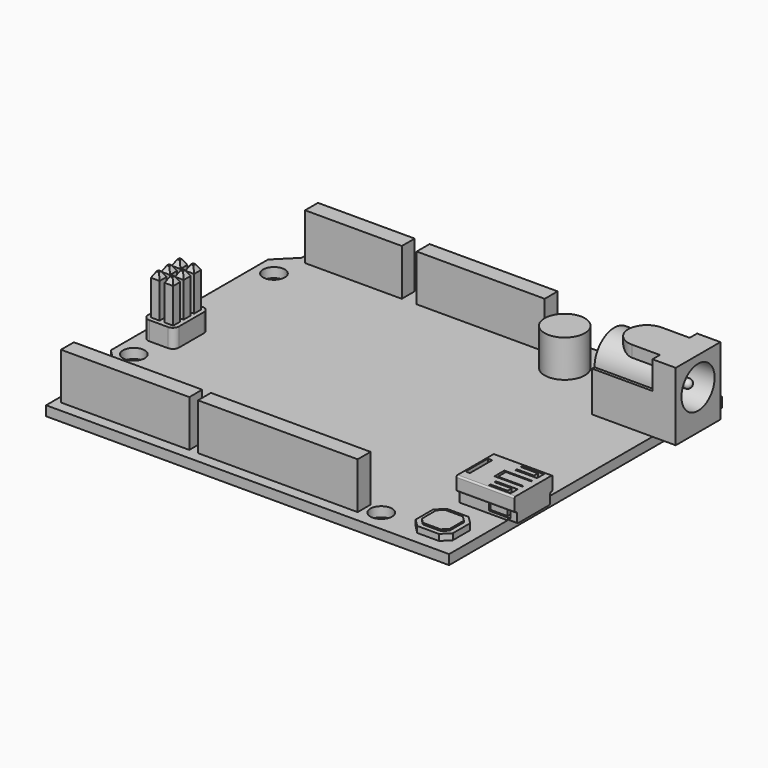
from build123d import *

# Parameters (mm, degrees)
F0_W           = 65
F0_H           = 55
F1_DEPTH       = 1.57
F3_DEPTH       = 1.57
F4_R           = 1.75
F5_DEPTH       = 1.571
F6_W           = 9
F6_H           = 11
F7_DEPTH       = 11
F7_DEPTH_BACK  = 3.75
F9_DEPTH       = 4.5
F10_R          = 4
F11_DEPTH      = 11
F12_W          = 1.25
F12_H          = 6.75
F13_DEPTH      = 11
F14_W          = 1.25
F14_H          = 2.25
F15_DEPTH      = 4.5010001
F15_DEPTH_BACK = 4.57
F16_R          = 3.3409090909
F17_DEPTH      = 10
F18_R          = 0.7
F19_DEPTH      = 9
F20_R          = 0.7
F21_W          = 7.7
F21_H          = 4
F22_DEPTH      = 7.86
F22_DEPTH_BACK = 1.5
F23_W          = 15.6
F23_H          = 2.6
F23_W_2        = 20.65
F23_W_3        = 20.7
F23_W_4        = 25.75
F24_DEPTH      = 7.5
F26_W          = 0.5
F26_H          = 1.75
F27_DEPTH      = 69.501
F25_W          = 0.7
F25_H          = 4.5
F25_W_2        = 4.1
F25_H_2        = 0.2
F28_DEPTH      = 3.6
F29_R          = 0.24999
F31_DEPTH      = 1
F33_DEPTH      = 0.25
F34_W          = 5
F34_H          = 7
F35_DEPTH      = 3
F36_W          = 1.4
F36_H          = 1.4
F37_DEPTH      = 6.5
F38_T1_DEPTH   = 5.8809639706
F38_T3_DEPTH   = 5.8809639706
F38_T5_DEPTH   = 5.8809639706
F38_T7_DEPTH   = 5.8809639706
F38_T9_DEPTH   = 5.8809639706
F39_R          = 1
F40_R          = 3.25
F41_DEPTH      = 6
F42_C1_SIZE2   = 0.5
F42_C1_SIZE    = 0.8660254038
F42_C2_SIZE2   = 0.5
F42_C2_SIZE    = 0.8660254038
F42_C3_SIZE2   = 0.5
F42_C3_SIZE    = 0.8660254038
F42_C4_SIZE2   = 0.5
F42_C4_SIZE    = 0.8660254038
F42_C5_SIZE2   = 0.5
F42_C5_SIZE    = 0.8660254038
F42_C6_SIZE2   = 0.5
F42_C6_SIZE    = 0.8660254038


# Not quite as in the source:
# - a fillet or chamfer that OpenCascade refuses, or shapes differently, is made with other operations: its cross-section is extruded or revolved along the edge and cut away or added
# - a fillet or chamfer is up to 0.001 mm smaller than in the source, because OpenCascade refuses the exact size


with BuildPart() as f1:
    # F0 (on Top) → F1 (new body)
    with BuildSketch(Plane.XY):
        Rectangle(F0_W, F0_H)
    extrude(amount=F1_DEPTH)

    # F2 (on face) → F3 (join, through all)
    with BuildSketch(Plane.XY.offset(1.57)):
        Polygon((-32.5, -13.7), (-32.5, 24), (-35.5, 20.9896013553), (-35.5, -10.6896013553), align=None)
    extrude(amount=-F3_DEPTH)

    # F4 (on face) → F5 (cut, through all)
    with BuildSketch(Plane.XY.offset(1.57)):
        with Locations((-32.55, 18.5)):
            Circle(F4_R)
        with Locations((-32.55, -9.75)):
            Circle(F4_R)
        with Locations((18.75, 24)):
            Circle(F4_R)
        with Locations((18.75, -24)):
            Circle(F4_R)
    extrude(amount=-F5_DEPTH, mode=Mode.SUBTRACT)

    # F6 (on face) → F7 (join, two sides)
    with BuildSketch(Plane.YZ.offset(32.5)) as f7_sk:
        with Locations((18, 7.07)):
            Rectangle(F6_W, F6_H)
    extrude(amount=-F7_DEPTH)
    extrude(f7_sk.sketch, amount=F7_DEPTH_BACK)

    # F8 (on face) → F9 (cut)
    with BuildSketch(Plane.XY.offset(12.57)):
        Polygon((21.5, 13.5), (32.5, 13.5), (32.5, 15), (28, 15), (25, 15), (25, 18), (25, 21), (28, 21), (32.5, 21), (32.5, 22.5), (21.5, 22.5), align=None)
        with BuildLine():
            ThreePointArc((25, 18), (25.8786796564, 20.1213203436), (28, 21))
            Line((28, 21), (25, 21))
            Line((25, 21), (25, 18))
        make_face()
        with BuildLine():
            Line((25, 15), (28, 15))
            ThreePointArc((28, 15), (25.8786796564, 15.8786796564), (25, 18))
            Line((25, 18), (25, 15))
        make_face()
    extrude(amount=-F9_DEPTH, mode=Mode.SUBTRACT)

    # F10 (on face) → F11 (join, through all)
    with BuildSketch(Plane(origin=(21.5, 0, 0), x_dir=(0, -1, 0), z_dir=(-1, 0, 0))):
        with Locations((-18, 8.07)):
            Circle(F10_R)
    extrude(amount=-F11_DEPTH)

    # F12 (on face) → F13 (cut, through all)
    with BuildSketch(Plane.XY.offset(12.57)):
        with Locations((22.125, 16.875)):
            Rectangle(F12_W, F12_H)
    extrude(amount=-F13_DEPTH, mode=Mode.SUBTRACT)

    # F14 (on face) → F15 (cut, two sides)
    with BuildSketch(Plane.XY.offset(8.07)) as f15_sk:
        with Locations((22.125, 21.375)):
            Rectangle(F14_W, F14_H)
    extrude(amount=F15_DEPTH, mode=Mode.SUBTRACT)
    extrude(f15_sk.sketch, amount=-F15_DEPTH_BACK, mode=Mode.SUBTRACT)

    # F16 (on face) → F17 (cut)
    with BuildSketch(Plane.YZ.offset(36.25)):
        with Locations((18, 7.9790909091)):
            Circle(F16_R)
    extrude(amount=-F17_DEPTH, mode=Mode.SUBTRACT)

    # F18 (on face) → F19 (join, through all)
    with BuildSketch(Plane.YZ.offset(26.25)):
        with Locations((18, 7.9790909091)):
            Circle(F18_R)
    extrude(amount=F19_DEPTH)

    # F20
    f20_edges = [f1.edges().sort_by_distance(p)[0] for p in [
        (35.25, 17.3, 7.979091),
    ]]
    fillet(f20_edges, radius=F20_R)

    # F21 (on face) → F22 (join, two sides)
    with BuildSketch(Plane.YZ.offset(32.5)) as f22_sk:
        with Locations((-12.35, 3.57)):
            Rectangle(F21_W, F21_H)
    extrude(amount=-F22_DEPTH)
    extrude(f22_sk.sketch, amount=F22_DEPTH_BACK)

    # F23 (on face) → F24 (join)
    with BuildSketch(Plane.XY.offset(1.57)):
        with Locations((-23.45, 24.45)):
            Rectangle(F23_W, F23_H)
        with Locations((-2.925, 24.45)):
            Rectangle(F23_W_2, F23_H)
        with Locations((-21.15, -24.45)):
            Rectangle(F23_W_3, F23_H)
        with Locations((3.475, -24.45)):
            Rectangle(F23_W_4, F23_H)
    extrude(amount=F24_DEPTH)

    # F26 (on face) → F27 (cut, through all)
    with BuildSketch(Plane.YZ.offset(34)):
        with Locations((-15.95, 2.445)):
            Rectangle(F26_W, F26_H)
        with Locations((-8.75, 2.445)):
            Rectangle(F26_W, F26_H)
    extrude(amount=-F27_DEPTH, mode=Mode.SUBTRACT)

    # F25 (on face) → F28 (cut, through all)
    with BuildSketch(Plane.XY.offset(5.57)):
        with Locations((25.19, -12.35)):
            Rectangle(F25_W, F25_H)
        with Locations((30.95, -11.45)):
            Rectangle(F25_W_2, F25_H_2)
        Polygon((28.9, -11.55), (28.9, -11.35), (28.5, -11.35), (28.5, -13.35), (28.9, -13.35), (28.9, -13.15), align=None)
        with Locations((30.95, -13.25)):
            Rectangle(F25_W_2, F25_H_2)
        Polygon((33, -9), (29.5, -9), (29.5, -9.3), (32.25, -9.3), (32.25, -10.1), (29.5, -10.1), (29.5, -10.4), (33, -10.4), align=None)
        Polygon((33, -14.3), (29.5, -14.3), (29.5, -14.6), (32.25, -14.6), (32.25, -15.4), (29.5, -15.4), (29.5, -15.7), (33, -15.7), align=None)
    extrude(amount=-F28_DEPTH, mode=Mode.SUBTRACT)

    # F29 (radius 0.25 in the source; OpenCascade refuses exactly that, so slightly less here)
    f29_edges = [f1.edges().sort_by_distance(p)[0] for p in [
        (29.32, -8.5, 5.57),
        (29.32, -16.2, 5.57),
        (33.5, -15.7, 3.32),
        (33.5, -9, 3.32),
        (33.25, -15.7, 1.57),
        (33.25, -9, 1.57),
        (29.32, -8.5, 3.32),
        (29.32, -16.2, 3.32),
        (24.64, -15.7, 2.445),
        (24.64, -9, 2.445),
    ]]
    fillet(f29_edges, radius=F29_R)

    # F30 (on face) → F31 (join)
    with BuildSketch(Plane.XY.offset(1.57)):
        Polygon((25.7625631329, -19.5251262658), (24.5251262658, -20.7625631329), (24.5251262658, -24.2625631329), (25.7625631329, -25.5), (29.2625631329, -25.5), (30.5, -24.2625631329), (30.5, -20.7625631329), (29.2625631329, -19.5251262658), align=None)
    extrude(amount=F31_DEPTH)

    # F32 (on face) → F33 (join)
    with BuildSketch(Plane.XY.offset(2.57)):
        Polygon((28.9519029611, -20.2751262658), (26.0732233047, -20.2751262658), (25.2751262658, -21.0732233047), (25.2751262658, -23.9519029611), (26.0732233047, -24.75), (28.9519029611, -24.75), (29.75, -23.9519029611), (29.75, -21.0732233047), align=None)
    extrude(amount=F33_DEPTH)

    # F34 (on face) → F35 (join)
    with BuildSketch(Plane.XY.offset(1.57)):
        with Locations((-31.75, -2.25)):
            Rectangle(F34_W, F34_H)
    extrude(amount=F35_DEPTH)

    # F36 (on face) → F37 (join)
    with BuildSketch(Plane.XY.offset(4.57)):
        with Locations((-32.85, -0.15)):
            Rectangle(F36_W, F36_H)
        with Locations((-30.65, -0.15)):
            Rectangle(F36_W, F36_H)
        with Locations((-32.85, -2.25)):
            Rectangle(F36_W, F36_H)
        with Locations((-30.65, -2.25)):
            Rectangle(F36_W, F36_H)
        with Locations((-32.85, -4.35)):
            Rectangle(F36_W, F36_H)
        with Locations((-30.65, -4.35)):
            Rectangle(F36_W, F36_H)
    extrude(amount=F37_DEPTH)

    # F38: chamfer of 0.5 x 0.8660254038 on 12 edges, made by hand

    # F38_s2 → F38_t1 (cut)
    with BuildSketch(Plane.XZ.offset(1.4095180147)):
        Polygon((-29.95, 10.2039745962), (-30.45, 11.07), (-29.95, 11.07), align=None)
        Polygon((-32.15, 10.2039745962), (-32.65, 11.07), (-32.15, 11.07), align=None)
    extrude(amount=F38_T1_DEPTH, mode=Mode.SUBTRACT)

    # F38_s4 → F38_t3 (cut)
    with BuildSketch(Plane.YZ.offset(-33.5904819853)):
        Polygon((-5.05, 10.2039745962), (-4.55, 11.07), (-5.05, 11.07), align=None)
        Polygon((-2.95, 10.2039745962), (-2.45, 11.07), (-2.95, 11.07), align=None)
        Polygon((-0.85, 10.2039745962), (-0.35, 11.07), (-0.85, 11.07), align=None)
    extrude(amount=F38_T3_DEPTH, mode=Mode.SUBTRACT)

    # F38_s6 → F38_t5 (cut)
    with BuildSketch(Plane.XZ.offset(-0.6904819853)):
        Polygon((-29.95, 10.2039745962), (-30.45, 11.07), (-29.95, 11.07), align=None)
        Polygon((-32.15, 10.2039745962), (-32.65, 11.07), (-32.15, 11.07), align=None)
    extrude(amount=F38_T5_DEPTH, mode=Mode.SUBTRACT)

    # F38_s8 → F38_t7 (cut)
    with BuildSketch(Plane.XZ.offset(-2.7904819853)):
        Polygon((-29.95, 10.2039745962), (-30.45, 11.07), (-29.95, 11.07), align=None)
        Polygon((-32.15, 10.2039745962), (-32.65, 11.07), (-32.15, 11.07), align=None)
    extrude(amount=F38_T7_DEPTH, mode=Mode.SUBTRACT)

    # F38_s10 → F38_t9 (cut)
    with BuildSketch(Plane.YZ.offset(-35.7904819853)):
        Polygon((-3.65, 10.2039745962), (-4.15, 11.07), (-3.65, 11.07), align=None)
        Polygon((-1.55, 10.2039745962), (-2.05, 11.07), (-1.55, 11.07), align=None)
        Polygon((0.55, 10.2039745962), (0.05, 11.07), (0.55, 11.07), align=None)
    extrude(amount=F38_T9_DEPTH, mode=Mode.SUBTRACT)

    # F39
    f39_edges = [f1.edges().sort_by_distance(p)[0] for p in [
        (-34.25, -5.75, 3.07),
        (-29.25, -5.75, 3.07),
        (-29.25, 1.25, 3.07),
        (-34.25, 1.25, 3.07),
    ]]
    fillet(f39_edges, radius=F39_R)

    # F40 (on face) → F41 (join)
    with BuildSketch(Plane.XY.offset(1.57)):
        with Locations((12.15, 21.25)):
            Circle(F40_R)
    extrude(amount=F41_DEPTH)

    # F42: chamfer of 0.5 x 0.8660254038 on 6 edges, made by hand

    # F42_c1
    f42_c1_edges = [f1.edges().sort_by_distance(p)[0] for p in [
        (-33.55, -4.35, 11.07),
    ]]
    f42_c1_side = f1.faces().sort_by_distance((-33.55, -4.35, 11.06))[0]
    chamfer(f42_c1_edges, length=F42_C1_SIZE, length2=F42_C1_SIZE2, reference=f42_c1_side)

    # F42_c2
    f42_c2_edges = [f1.edges().sort_by_distance(p)[0] for p in [
        (-31.35, -4.35, 11.07),
    ]]
    f42_c2_side = f1.faces().sort_by_distance((-31.35, -4.35, 11.06))[0]
    chamfer(f42_c2_edges, length=F42_C2_SIZE, length2=F42_C2_SIZE2, reference=f42_c2_side)

    # F42_c3
    f42_c3_edges = [f1.edges().sort_by_distance(p)[0] for p in [
        (-33.55, -2.25, 11.07),
    ]]
    f42_c3_side = f1.faces().sort_by_distance((-33.55, -2.25, 11.06))[0]
    chamfer(f42_c3_edges, length=F42_C3_SIZE, length2=F42_C3_SIZE2, reference=f42_c3_side)

    # F42_c4
    f42_c4_edges = [f1.edges().sort_by_distance(p)[0] for p in [
        (-33.55, -0.15, 11.07),
    ]]
    f42_c4_side = f1.faces().sort_by_distance((-33.55, -0.15, 11.06))[0]
    chamfer(f42_c4_edges, length=F42_C4_SIZE, length2=F42_C4_SIZE2, reference=f42_c4_side)

    # F42_c5
    f42_c5_edges = [f1.edges().sort_by_distance(p)[0] for p in [
        (-31.35, -2.25, 11.07),
    ]]
    f42_c5_side = f1.faces().sort_by_distance((-31.35, -2.25, 11.06))[0]
    chamfer(f42_c5_edges, length=F42_C5_SIZE, length2=F42_C5_SIZE2, reference=f42_c5_side)

    # F42_c6
    f42_c6_edges = [f1.edges().sort_by_distance(p)[0] for p in [
        (-31.35, -0.15, 11.07),
    ]]
    f42_c6_side = f1.faces().sort_by_distance((-31.35, -0.15, 11.06))[0]
    chamfer(f42_c6_edges, length=F42_C6_SIZE, length2=F42_C6_SIZE2, reference=f42_c6_side)


solid = f1.part
